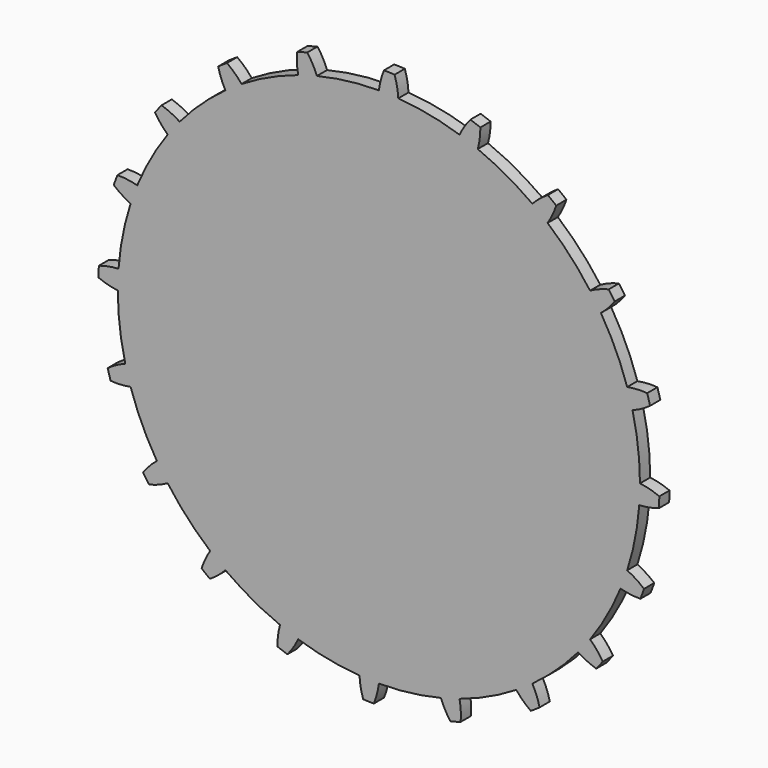
from build123d import *

# Parameters (mm, degrees)
F3_DEPTH      = 0.33
F3_DEPTH_BACK = 0.33


with BuildPart() as f3:
    # F2 (on Front) → F3 (new body, two sides)
    with BuildSketch(Plane.XZ) as f3_sk:
        with BuildLine():
            ThreePointArc((13.427331249, -0.9997678629), (13.4552046036, -0.5002292714), (13.4645, 0))
            ThreePointArc((13.4645, 0), (13.4644999955, 0.0003469704), (13.4644999821, 0.0006939409))
            ThreePointArc((13.4644999821, 0.0006939409), (13.3677602926, 1.6111315933), (13.0790961409, 3.1984378043))
            ThreePointArc((13.0790961409, 3.1984378043), (12.9511444719, 3.68247432), (12.8052860071, 4.1614192922))
            ThreePointArc((12.8052860071, 4.1614192922), (12.215628492, 5.6631423075), (11.4505879751, 7.0835580943))
            ThreePointArc((11.4505879751, 7.0835580943), (11.1793231973, 7.5043649366), (10.8926014181, 7.9147959289))
            ThreePointArc((10.8926014181, 7.9147959289), (9.8677458634, 9.1608051953), (8.7012164773, 10.275290364))
            ThreePointArc((8.7012164773, 10.275290364), (8.3131918771, 10.5916760271), (7.913673109, 10.8934171945))
            ThreePointArc((7.913673109, 10.8934171945), (6.553939517, 11.7617446434), (5.1001092858, 12.4612056208))
            ThreePointArc((5.1001092858, 12.4612056208), (4.6333074147, 12.6422000716), (4.1600993383, 12.8057148862))
            ThreePointArc((4.1600993383, 12.8057148862), (2.5985879067, 13.211362577), (0.9997678629, 13.427331249))
            ThreePointArc((0.9997678629, 13.427331249), (0.4998825403, 13.4552174897), (-0.0006939409, 13.4644999821))
            ThreePointArc((-0.0006939409, 13.4644999821), (-1.6111315933, 13.3677602926), (-3.1984378043, 13.0790961409))
            ThreePointArc((-3.1984378043, 13.0790961409), (-3.68247432, 12.9511444719), (-4.1614192922, 12.8052860071))
            ThreePointArc((-4.1614192922, 12.8052860071), (-5.6631423075, 12.215628492), (-7.0835580943, 11.4505879751))
            ThreePointArc((-7.0835580943, 11.4505879751), (-7.5043649366, 11.1793231973), (-7.9147959289, 10.8926014181))
            ThreePointArc((-7.9147959289, 10.8926014181), (-9.1608051953, 9.8677458634), (-10.275290364, 8.7012164773))
            ThreePointArc((-10.275290364, 8.7012164773), (-10.5916760271, 8.3131918771), (-10.8934171945, 7.913673109))
            ThreePointArc((-10.8934171945, 7.913673109), (-11.7617446434, 6.553939517), (-12.4612056208, 5.1001092858))
            ThreePointArc((-12.4612056208, 5.1001092858), (-12.6422000716, 4.6333074147), (-12.8057148862, 4.1600993383))
            ThreePointArc((-12.8057148862, 4.1600993383), (-13.211362577, 2.5985879067), (-13.427331249, 0.9997678629))
            ThreePointArc((-13.427331249, 0.9997678629), (-13.4552174897, 0.4998825403), (-13.4644999821, -0.0006939409))
            ThreePointArc((-13.4644999821, -0.0006939409), (-13.3677602926, -1.6111315933), (-13.0790961409, -3.1984378043))
            ThreePointArc((-13.0790961409, -3.1984378043), (-12.9511444719, -3.68247432), (-12.8052860071, -4.1614192922))
            ThreePointArc((-12.8052860071, -4.1614192922), (-12.215628492, -5.6631423075), (-11.4505879751, -7.0835580943))
            ThreePointArc((-11.4505879751, -7.0835580943), (-11.1793231973, -7.5043649366), (-10.8926014181, -7.9147959289))
            ThreePointArc((-10.8926014181, -7.9147959289), (-9.8677458634, -9.1608051953), (-8.7012164773, -10.275290364))
            ThreePointArc((-8.7012164773, -10.275290364), (-8.3131918771, -10.5916760271), (-7.913673109, -10.8934171945))
            ThreePointArc((-7.913673109, -10.8934171945), (-6.553939517, -11.7617446434), (-5.1001092858, -12.4612056208))
            ThreePointArc((-5.1001092858, -12.4612056208), (-4.6333074147, -12.6422000716), (-4.1600993383, -12.8057148862))
            ThreePointArc((-4.1600993383, -12.8057148862), (-2.5985879067, -13.211362577), (-0.9997678629, -13.427331249))
            ThreePointArc((-0.9997678629, -13.427331249), (-0.4998825403, -13.4552174897), (0.0006939409, -13.4644999821))
            ThreePointArc((0.0006939409, -13.4644999821), (1.6111315933, -13.3677602926), (3.1984378043, -13.0790961409))
            ThreePointArc((3.1984378043, -13.0790961409), (3.68247432, -12.9511444719), (4.1614192922, -12.8052860071))
            ThreePointArc((4.1614192922, -12.8052860071), (5.6631423075, -12.215628492), (7.0835580943, -11.4505879751))
            ThreePointArc((7.0835580943, -11.4505879751), (7.5043649366, -11.1793231973), (7.9147959289, -10.8926014181))
            ThreePointArc((7.9147959289, -10.8926014181), (9.1608051953, -9.8677458634), (10.275290364, -8.7012164773))
            ThreePointArc((10.275290364, -8.7012164773), (10.5916760271, -8.3131918771), (10.8934171945, -7.913673109))
            ThreePointArc((10.8934171945, -7.913673109), (11.7617446434, -6.553939517), (12.4612056208, -5.1001092858))
            ThreePointArc((12.4612056208, -5.1001092858), (12.6422000716, -4.6333074147), (12.8057148862, -4.1600993383))
            ThreePointArc((12.8057148862, -4.1600993383), (13.211362577, -2.5985879067), (13.427331249, -0.9997678629))
        make_face()
        with BuildLine():
            ThreePointArc((13.4644999821, 0.0006939409), (13.4644999955, 0.0003469704), (13.4645, 0))
            ThreePointArc((13.4645, 0), (13.4552046036, -0.5002292714), (13.427331249, -0.9997678629))
            ThreePointArc((13.427331249, -0.9997678629), (13.9409777525, -0.9393106229), (14.4417920292, -0.8101871604))
            ThreePointArc((14.4417920292, -0.8101871604), (14.4545280835, -0.5370085042), (14.4620971963, -0.2636378879))
            ThreePointArc((14.4620971963, -0.2636378879), (13.9722445576, -0.0977095878), (13.4644999821, 0.0006939409))
        make_face()
        with BuildLine():
            ThreePointArc((12.8052860071, 4.1614192922), (12.9511444719, 3.68247432), (13.0790961409, 3.1984378043))
            ThreePointArc((13.0790961409, 3.1984378043), (13.5489206805, 3.4146615549), (13.9853220175, 3.692225388))
            ThreePointArc((13.9853220175, 3.692225388), (13.9130178777, 3.9559693863), (13.8357403655, 4.2182992767))
            ThreePointArc((13.8357403655, 4.2182992767), (13.3185881569, 4.2247336777), (12.8052860071, 4.1614192922))
        make_face()
        with BuildLine():
            ThreePointArc((13.6728031901, -4.7197683392), (13.2582003107, -4.410588358), (12.8057148862, -4.1600993383))
            ThreePointArc((12.8057148862, -4.1600993383), (12.6422000716, -4.6333074147), (12.4612056208, -5.1001092858))
            ThreePointArc((12.4612056208, -5.1001092858), (12.9683947895, -5.2013365325), (13.4845988152, -5.2332929446))
            ThreePointArc((13.4845988152, -5.2332929446), (13.5811283699, -4.9774202606), (13.6728031901, -4.7197683392))
        make_face()
        with BuildLine():
            ThreePointArc((10.8926014181, 7.9147959289), (11.1793231973, 7.5043649366), (11.4505879751, 7.0835580943))
            ThreePointArc((11.4505879751, 7.0835580943), (11.8306008514, 7.4343828685), (12.1598712453, 7.8332171901))
            ThreePointArc((12.1598712453, 7.8332171901), (12.0096045443, 8.0617094303), (11.8550448685, 8.2873199175))
            ThreePointArc((11.8550448685, 8.2873199175), (11.3612155514, 8.1336305754), (10.8926014181, 7.9147959289))
        make_face()
        with BuildLine():
            ThreePointArc((11.5451199436, -8.7138949808), (11.246351042, -8.2917280094), (10.8934171945, -7.913673109))
            ThreePointArc((10.8934171945, -7.913673109), (10.5916760271, -8.3131918771), (10.275290364, -8.7012164773))
            ThreePointArc((10.275290364, -8.7012164773), (10.7263749885, -8.9542193824), (11.2074391164, -9.1441275528))
            ThreePointArc((11.2074391164, -9.1441275528), (11.3783131861, -8.9306074423), (11.5451199436, -8.7138949808))
        make_face()
        with BuildLine():
            ThreePointArc((7.913673109, 10.8934171945), (8.3131918771, 10.5916760271), (8.7012164773, 10.275290364))
            ThreePointArc((8.7012164773, 10.275290364), (8.9542193824, 10.7263749885), (9.1441275528, 11.2074391164))
            ThreePointArc((9.1441275528, 11.2074391164), (8.9306074423, 11.3783131861), (8.7138949808, 11.5451199436))
            ThreePointArc((8.7138949808, 11.5451199436), (8.2917280094, 11.246351042), (7.913673109, 10.8934171945))
        make_face()
        with BuildLine():
            ThreePointArc((8.2873199175, -11.8550448685), (8.1336305754, -11.3612155514), (7.9147959289, -10.8926014181))
            ThreePointArc((7.9147959289, -10.8926014181), (7.5043649366, -11.1793231973), (7.0835580943, -11.4505879751))
            ThreePointArc((7.0835580943, -11.4505879751), (7.4343828685, -11.8306008514), (7.8332171901, -12.1598712453))
            ThreePointArc((7.8332171901, -12.1598712453), (8.0617094303, -12.0096045443), (8.2873199175, -11.8550448685))
        make_face()
        with BuildLine():
            ThreePointArc((4.1600993383, 12.8057148862), (4.6333074147, 12.6422000716), (5.1001092858, 12.4612056208))
            ThreePointArc((5.1001092858, 12.4612056208), (5.2013365325, 12.9683947895), (5.2332929446, 13.4845988152))
            ThreePointArc((5.2332929446, 13.4845988152), (4.9774202606, 13.5811283699), (4.7197683392, 13.6728031901))
            ThreePointArc((4.7197683392, 13.6728031901), (4.410588358, 13.2582003107), (4.1600993383, 12.8057148862))
        make_face()
        with BuildLine():
            ThreePointArc((4.2182992767, -13.8357403655), (4.2247336777, -13.3185881569), (4.1614192922, -12.8052860071))
            ThreePointArc((4.1614192922, -12.8052860071), (3.68247432, -12.9511444719), (3.1984378043, -13.0790961409))
            ThreePointArc((3.1984378043, -13.0790961409), (3.4146615549, -13.5489206805), (3.692225388, -13.9853220175))
            ThreePointArc((3.692225388, -13.9853220175), (3.9559693863, -13.9130178777), (4.2182992767, -13.8357403655))
        make_face()
        with BuildLine():
            ThreePointArc((-0.0006939409, 13.4644999821), (0.4998825403, 13.4552174897), (0.9997678629, 13.427331249))
            ThreePointArc((0.9997678629, 13.427331249), (0.9393106229, 13.9409777525), (0.8101871604, 14.4417920292))
            ThreePointArc((0.8101871604, 14.4417920292), (0.5370085042, 14.4545280835), (0.2636378879, 14.4620971963))
            ThreePointArc((0.2636378879, 14.4620971963), (0.0977095878, 13.9722445576), (-0.0006939409, 13.4644999821))
        make_face()
        with BuildLine():
            ThreePointArc((-0.2636378879, -14.4620971963), (-0.0977095878, -13.9722445576), (0.0006939409, -13.4644999821))
            ThreePointArc((0.0006939409, -13.4644999821), (-0.4998825403, -13.4552174897), (-0.9997678629, -13.427331249))
            ThreePointArc((-0.9997678629, -13.427331249), (-0.9393106229, -13.9409777525), (-0.8101871604, -14.4417920292))
            ThreePointArc((-0.8101871604, -14.4417920292), (-0.5370085042, -14.4545280835), (-0.2636378879, -14.4620971963))
        make_face()
        with BuildLine():
            ThreePointArc((-4.1614192922, 12.8052860071), (-3.68247432, 12.9511444719), (-3.1984378043, 13.0790961409))
            ThreePointArc((-3.1984378043, 13.0790961409), (-3.4146615549, 13.5489206805), (-3.692225388, 13.9853220175))
            ThreePointArc((-3.692225388, 13.9853220175), (-3.9559693863, 13.9130178777), (-4.2182992767, 13.8357403655))
            ThreePointArc((-4.2182992767, 13.8357403655), (-4.2247336777, 13.3185881569), (-4.1614192922, 12.8052860071))
        make_face()
        with BuildLine():
            ThreePointArc((-4.7197683392, -13.6728031901), (-4.410588358, -13.2582003107), (-4.1600993383, -12.8057148862))
            ThreePointArc((-4.1600993383, -12.8057148862), (-4.6333074147, -12.6422000716), (-5.1001092858, -12.4612056208))
            ThreePointArc((-5.1001092858, -12.4612056208), (-5.2013365325, -12.9683947895), (-5.2332929446, -13.4845988152))
            ThreePointArc((-5.2332929446, -13.4845988152), (-4.9774202606, -13.5811283699), (-4.7197683392, -13.6728031901))
        make_face()
        with BuildLine():
            ThreePointArc((-7.9147959289, 10.8926014181), (-7.5043649366, 11.1793231973), (-7.0835580943, 11.4505879751))
            ThreePointArc((-7.0835580943, 11.4505879751), (-7.4343828685, 11.8306008514), (-7.8332171901, 12.1598712453))
            ThreePointArc((-7.8332171901, 12.1598712453), (-8.0617094303, 12.0096045443), (-8.2873199175, 11.8550448685))
            ThreePointArc((-8.2873199175, 11.8550448685), (-8.1336305754, 11.3612155514), (-7.9147959289, 10.8926014181))
        make_face()
        with BuildLine():
            ThreePointArc((-8.7138949808, -11.5451199436), (-8.2917280094, -11.246351042), (-7.913673109, -10.8934171945))
            ThreePointArc((-7.913673109, -10.8934171945), (-8.3131918771, -10.5916760271), (-8.7012164773, -10.275290364))
            ThreePointArc((-8.7012164773, -10.275290364), (-8.9542193824, -10.7263749885), (-9.1441275528, -11.2074391164))
            ThreePointArc((-9.1441275528, -11.2074391164), (-8.9306074423, -11.3783131861), (-8.7138949808, -11.5451199436))
        make_face()
        with BuildLine():
            ThreePointArc((-10.8934171945, 7.913673109), (-10.5916760271, 8.3131918771), (-10.275290364, 8.7012164773))
            ThreePointArc((-10.275290364, 8.7012164773), (-10.7263749885, 8.9542193824), (-11.2074391164, 9.1441275528))
            ThreePointArc((-11.2074391164, 9.1441275528), (-11.3783131861, 8.9306074423), (-11.5451199436, 8.7138949808))
            ThreePointArc((-11.5451199436, 8.7138949808), (-11.246351042, 8.2917280094), (-10.8934171945, 7.913673109))
        make_face()
        with BuildLine():
            ThreePointArc((-11.8550448685, -8.2873199175), (-11.3612155514, -8.1336305754), (-10.8926014181, -7.9147959289))
            ThreePointArc((-10.8926014181, -7.9147959289), (-11.1793231973, -7.5043649366), (-11.4505879751, -7.0835580943))
            ThreePointArc((-11.4505879751, -7.0835580943), (-11.8306008514, -7.4343828685), (-12.1598712453, -7.8332171901))
            ThreePointArc((-12.1598712453, -7.8332171901), (-12.0096045443, -8.0617094303), (-11.8550448685, -8.2873199175))
        make_face()
        with BuildLine():
            ThreePointArc((-12.8057148862, 4.1600993383), (-12.6422000716, 4.6333074147), (-12.4612056208, 5.1001092858))
            ThreePointArc((-12.4612056208, 5.1001092858), (-12.9683947895, 5.2013365325), (-13.4845988152, 5.2332929446))
            ThreePointArc((-13.4845988152, 5.2332929446), (-13.5811283699, 4.9774202606), (-13.6728031901, 4.7197683392))
            ThreePointArc((-13.6728031901, 4.7197683392), (-13.2582003107, 4.410588358), (-12.8057148862, 4.1600993383))
        make_face()
        with BuildLine():
            ThreePointArc((-13.8357403655, -4.2182992767), (-13.3185881569, -4.2247336777), (-12.8052860071, -4.1614192922))
            ThreePointArc((-12.8052860071, -4.1614192922), (-12.9511444719, -3.68247432), (-13.0790961409, -3.1984378043))
            ThreePointArc((-13.0790961409, -3.1984378043), (-13.5489206805, -3.4146615549), (-13.9853220175, -3.692225388))
            ThreePointArc((-13.9853220175, -3.692225388), (-13.9130178777, -3.9559693863), (-13.8357403655, -4.2182992767))
        make_face()
        with BuildLine():
            ThreePointArc((-13.4644999821, -0.0006939409), (-13.4552174897, 0.4998825403), (-13.427331249, 0.9997678629))
            ThreePointArc((-13.427331249, 0.9997678629), (-13.9409777525, 0.9393106229), (-14.4417920292, 0.8101871604))
            ThreePointArc((-14.4417920292, 0.8101871604), (-14.4545280835, 0.5370085042), (-14.4620971963, 0.2636378879))
            ThreePointArc((-14.4620971963, 0.2636378879), (-13.9722445576, 0.0977095878), (-13.4644999821, -0.0006939409))
        make_face()
    extrude(amount=F3_DEPTH)
    extrude(f3_sk.sketch, amount=-F3_DEPTH_BACK)


solid = f3.part
